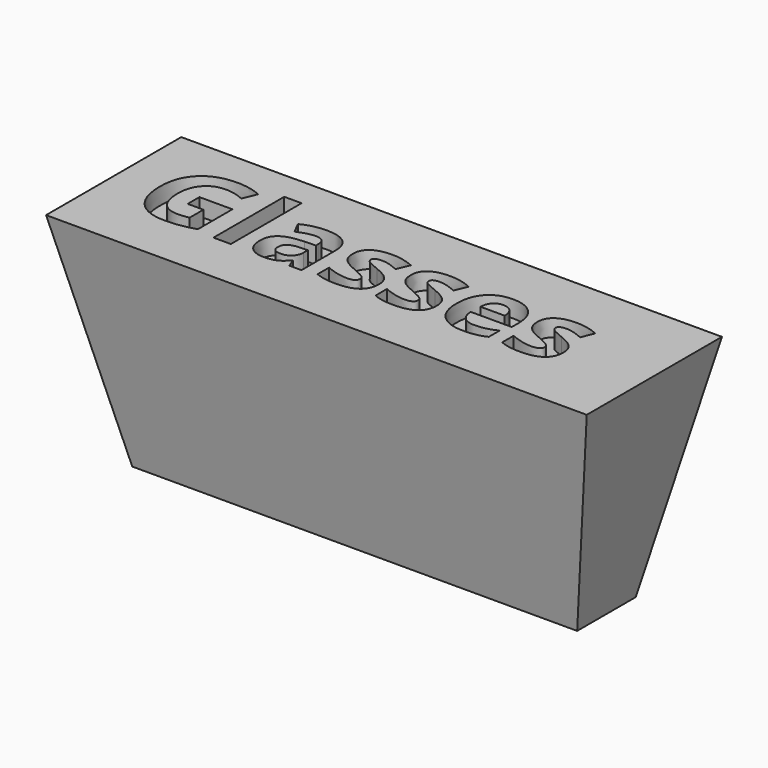
from build123d import *

# Parameters (mm, degrees)
F0_W         = 2438.4
F0_H         = 762
F1_DEPTH     = 1016
F1_TAPER     = 12
F2_TEXT_SIZE = 525.1310972704
F3_DEPTH     = 76.2


# Not quite as in the source:
# - Text() gives the source's letters only with a copy of the font that has no kerning and outlines rounded to 1/6400 em; it was checked with that copy


with BuildPart() as f1:
    # F0 (on Top) → F1 (new body)
    with BuildSketch(Plane.XY):
        Rectangle(F0_W, F0_H)
    extrude(amount=-F1_DEPTH, taper=F1_TAPER)

    # F2 (on face) → F3 (cut)
    with BuildSketch(Plane.XY):
        with Locations((-1072.7508068085, -146.9879001379)):
            Text('Glasses', F2_TEXT_SIZE, font='Open Sans', font_style=FontStyle.BOLD, text_align=(TextAlign.LEFT, TextAlign.BOTTOM))
    extrude(amount=-F3_DEPTH, mode=Mode.SUBTRACT)


solid = f1.part
